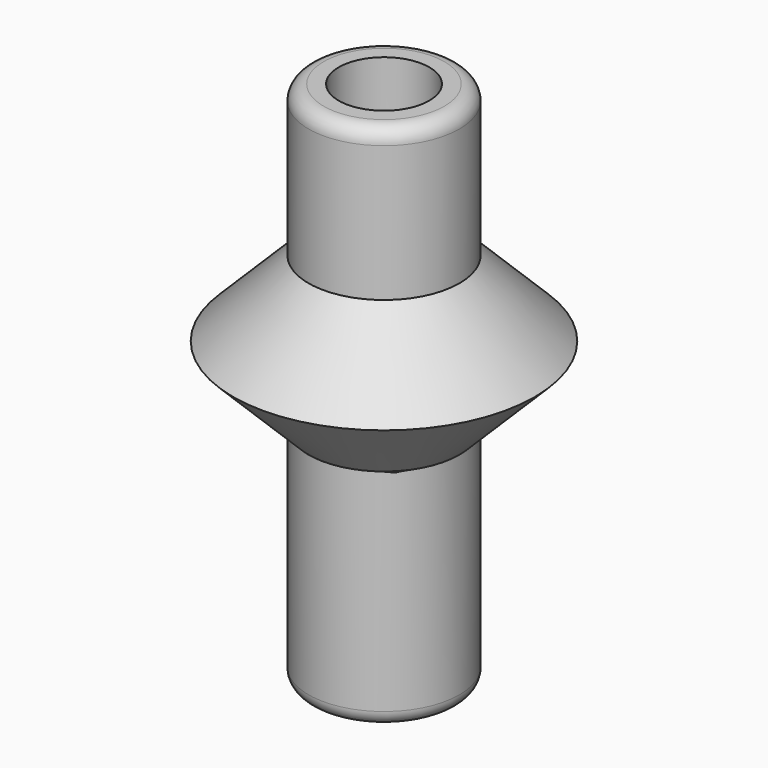
from build123d import *

# Parameters (mm, degrees)
F0_R         = 12.7
F1_DEPTH     = 38.1
F2_R         = 25.4
F2_R_2       = 12.7
F3_DEPTH     = 12.7
F4_R         = 2.54
F5_T1_DEPTH  = 10.7763073453
F5_T3_DEPTH  = 10.7763073453
F5_T9_DEPTH  = 23.4763073453
F5_S10_R     = 12.7
F5_T11_DEPTH = 14
F5_T15_DEPTH = 23.4763073453
F5_S16_R     = 12.7
F5_T17_DEPTH = 14
F5_T24_DEPTH = 23.4763073453
F5_S25_R     = 12.7
F5_T26_DEPTH = 14
F5_T30_DEPTH = 23.4763073453
F5_S31_R     = 12.7
F5_T32_DEPTH = 14
F5_T39_DEPTH = 23.4763073453
F5_S40_R     = 12.7
F5_T41_DEPTH = 14
F5_T45_DEPTH = 23.4763073453
F5_S46_R     = 12.7
F5_T47_DEPTH = 14
F5_T54_DEPTH = 23.4763073453
F5_S55_R     = 12.7
F5_T56_DEPTH = 14
F5_T60_DEPTH = 23.4763073453
F5_S61_R     = 12.7
F5_T62_DEPTH = 14
F8_R         = 12.7
F8_R_2       = 7.62
F9_DEPTH     = 25.4
F10_R        = 2.54
F11_DEPTH    = 25.4
F12_SIZE     = 12.69999


# Not quite as in the source:
# - a fillet or chamfer that OpenCascade refuses, or shapes differently, is made with other operations: its cross-section is extruded or revolved along the edge and cut away or added
# - a fillet or chamfer is up to 0.001 mm smaller than in the source, because OpenCascade refuses the exact size


with BuildPart() as f1:
    # F0 (on Top) → F1 (new body)
    with BuildSketch(Plane.XY):
        Circle(F0_R)
        with BuildLine():
            ThreePointArc((5.3881536726, 5.3881536726), (7.0399620377, 2.9160477546), (7.62, 0))
            ThreePointArc((7.62, 0), (7.0399620377, -2.9160477546), (5.3881536726, -5.3881536726))
            ThreePointArc((5.3881536726, -5.3881536726), (0, -7.62), (-5.3881536726, -5.3881536726))
            ThreePointArc((-5.3881536726, -5.3881536726), (-7.62, 0), (-5.3881536726, 5.3881536726))
            ThreePointArc((-5.3881536726, 5.3881536726), (0, 7.62), (5.3881536726, 5.3881536726))
        make_face(mode=Mode.SUBTRACT)
        with BuildLine():
            ThreePointArc((-5.3881536726, -5.3881536726), (0, -7.62), (5.3881536726, -5.3881536726))
            Line((5.3881536726, -5.3881536726), (-5.3881536726, -5.3881536726))
        make_face()
        with BuildLine():
            Line((-5.3881536726, -5.3881536726), (-5.3881536726, 5.3881536726))
            ThreePointArc((-5.3881536726, 5.3881536726), (-7.62, 0), (-5.3881536726, -5.3881536726))
        make_face()
        with BuildLine():
            ThreePointArc((5.3881536726, -5.3881536726), (7.0399620377, -2.9160477546), (7.62, 0))
            ThreePointArc((7.62, 0), (7.0399620377, 2.9160477546), (5.3881536726, 5.3881536726))
            Line((5.3881536726, 5.3881536726), (5.3881536726, -5.3881536726))
        make_face()
        with BuildLine():
            Line((-5.3881536726, 5.3881536726), (5.3881536726, 5.3881536726))
            ThreePointArc((5.3881536726, 5.3881536726), (0, 7.62), (-5.3881536726, 5.3881536726))
        make_face()
    extrude(amount=F1_DEPTH)

    # F4
    f4_edges = [f1.edges().sort_by_distance(p)[0] for p in [
        (-12.7, 0, 0),
    ]]
    fillet(f4_edges, radius=F4_R)

    # F5: fillet of radius 5.08 on 4 edges, made by hand

    # F5_s2 → F5_t1 (cut)
    with BuildSketch(Plane.XZ.offset(-5.3881536726)):
        with BuildLine():
            ThreePointArc((10.4681536726, 38.1), (6.8760512242, 36.6121024484), (5.3881536726, 33.02))
            Line((5.3881536726, 33.02), (5.3881536726, 38.1))
            Line((5.3881536726, 38.1), (10.4681536726, 38.1))
        make_face()
        with BuildLine():
            ThreePointArc((-10.4681536726, 38.1), (-6.8760512242, 36.6121024484), (-5.3881536726, 33.02))
            Line((-5.3881536726, 33.02), (-5.3881536726, 38.1))
            Line((-5.3881536726, 38.1), (-10.4681536726, 38.1))
        make_face()
    extrude(amount=F5_T1_DEPTH, mode=Mode.SUBTRACT)

    # F5_s4 → F5_t3 (cut)
    with BuildSketch(Plane.YZ.offset(-5.3881536726)):
        with BuildLine():
            ThreePointArc((-10.4681536726, 38.1), (-6.8760512242, 36.6121024484), (-5.3881536726, 33.02))
            Line((-5.3881536726, 33.02), (-5.3881536726, 38.1))
            Line((-5.3881536726, 38.1), (-10.4681536726, 38.1))
        make_face()
        with BuildLine():
            ThreePointArc((10.4681536726, 38.1), (6.8760512242, 36.6121024484), (5.3881536726, 33.02))
            Line((5.3881536726, 33.02), (5.3881536726, 38.1))
            Line((5.3881536726, 38.1), (10.4681536726, 38.1))
        make_face()
    extrude(amount=F5_T3_DEPTH, mode=Mode.SUBTRACT)


with BuildPart() as f3:
    # F2 (on face) → F3 (new body)
    with BuildSketch(Plane.XY.offset(38.1)):
        Circle(F2_R)
        Circle(F2_R_2, mode=Mode.SUBTRACT)
    extrude(amount=F3_DEPTH)

    # F6: F3 across face


with BuildPart() as f5_tool7:
    # F5_s8 → F5_t9 (new body)
    with BuildSketch(Plane.YZ.offset(-5.3881536726)):
        with BuildLine():
            ThreePointArc((10.4681536726, 38.1), (6.8760512242, 36.6121024484), (5.3881536726, 33.02))
            Line((5.3881536726, 33.02), (5.3881536726, 38.1))
            Line((5.3881536726, 38.1), (10.4681536726, 38.1))
        make_face()
    extrude(amount=F5_T9_DEPTH)

    # F5_s10 → F5_t11 (intersect, symmetric)
    with BuildSketch(Plane.XY.offset(35.6)):
        Circle(F5_S10_R)
    extrude(amount=F5_T11_DEPTH, both=True, mode=Mode.INTERSECT)

    split(bisect_by=Plane.YZ.offset(5.3881536726), keep=Keep.TOP)


with BuildPart() as f5_tool13:
    # F5_s14 → F5_t15 (new body)
    with BuildSketch(Plane.XZ.offset(-18.0881536726)):
        with BuildLine():
            ThreePointArc((10.4681536726, 38.1), (6.8760512242, 36.6121024484), (5.3881536726, 33.02))
            Line((5.3881536726, 33.02), (5.3881536726, 38.1))
            Line((5.3881536726, 38.1), (10.4681536726, 38.1))
        make_face()
    extrude(amount=F5_T15_DEPTH)

    # F5_s16 → F5_t17 (intersect, symmetric)
    with BuildSketch(Plane.XY.offset(35.6)):
        Circle(F5_S16_R)
    extrude(amount=F5_T17_DEPTH, both=True, mode=Mode.INTERSECT)

    split(bisect_by=Plane.XZ.offset(-5.3881536726), keep=Keep.BOTTOM)


with BuildPart() as f5_tool7_1:
    add(f5_tool7.part)

    # F5_t19: intersect F5_tool13
    add(f5_tool13.part, mode=Mode.INTERSECT)


with BuildPart() as f1_1:
    add(f1.part)

    # F5_t5: cut F5_tool7
    add(f5_tool7_1.part, mode=Mode.SUBTRACT)


with BuildPart() as f5_tool22:
    # F5_s23 → F5_t24 (new body)
    with BuildSketch(Plane.YZ.offset(18.0881536726)):
        with BuildLine():
            ThreePointArc((-10.4681536726, 38.1), (-6.8760512242, 36.6121024484), (-5.3881536726, 33.02))
            Line((-5.3881536726, 33.02), (-5.3881536726, 38.1))
            Line((-5.3881536726, 38.1), (-10.4681536726, 38.1))
        make_face()
    extrude(amount=-F5_T24_DEPTH)

    # F5_s25 → F5_t26 (intersect, symmetric)
    with BuildSketch(Plane.XY.offset(35.6)):
        Circle(F5_S25_R)
    extrude(amount=F5_T26_DEPTH, both=True, mode=Mode.INTERSECT)

    split(bisect_by=Plane.YZ.offset(5.3881536726), keep=Keep.TOP)


with BuildPart() as f5_tool28:
    # F5_s29 → F5_t30 (new body)
    with BuildSketch(Plane.XZ.offset(-5.3881536726)):
        with BuildLine():
            ThreePointArc((10.4681536726, 38.1), (6.8760512242, 36.6121024484), (5.3881536726, 33.02))
            Line((5.3881536726, 33.02), (5.3881536726, 38.1))
            Line((5.3881536726, 38.1), (10.4681536726, 38.1))
        make_face()
    extrude(amount=F5_T30_DEPTH)

    # F5_s31 → F5_t32 (intersect, symmetric)
    with BuildSketch(Plane.XY.offset(35.6)):
        Circle(F5_S31_R)
    extrude(amount=F5_T32_DEPTH, both=True, mode=Mode.INTERSECT)

    split(bisect_by=Plane.XZ.offset(5.3881536726), keep=Keep.TOP)


with BuildPart() as f5_tool22_1:
    add(f5_tool22.part)

    # F5_t34: intersect F5_tool28
    add(f5_tool28.part, mode=Mode.INTERSECT)


with BuildPart() as f1_2:
    add(f1_1.part)

    # F5_t20: cut F5_tool22
    add(f5_tool22_1.part, mode=Mode.SUBTRACT)


with BuildPart() as f5_tool37:
    # F5_s38 → F5_t39 (new body)
    with BuildSketch(Plane.YZ.offset(5.3881536726)):
        with BuildLine():
            ThreePointArc((-10.4681536726, 38.1), (-6.8760512242, 36.6121024484), (-5.3881536726, 33.02))
            Line((-5.3881536726, 33.02), (-5.3881536726, 38.1))
            Line((-5.3881536726, 38.1), (-10.4681536726, 38.1))
        make_face()
    extrude(amount=-F5_T39_DEPTH)

    # F5_s40 → F5_t41 (intersect, symmetric)
    with BuildSketch(Plane.XY.offset(35.6)):
        Circle(F5_S40_R)
    extrude(amount=F5_T41_DEPTH, both=True, mode=Mode.INTERSECT)

    split(bisect_by=Plane.YZ.offset(-5.3881536726), keep=Keep.BOTTOM)


with BuildPart() as f5_tool43:
    # F5_s44 → F5_t45 (new body)
    with BuildSketch(Plane.XZ.offset(18.0881536726)):
        with BuildLine():
            ThreePointArc((-10.4681536726, 38.1), (-6.8760512242, 36.6121024484), (-5.3881536726, 33.02))
            Line((-5.3881536726, 33.02), (-5.3881536726, 38.1))
            Line((-5.3881536726, 38.1), (-10.4681536726, 38.1))
        make_face()
    extrude(amount=-F5_T45_DEPTH)

    # F5_s46 → F5_t47 (intersect, symmetric)
    with BuildSketch(Plane.XY.offset(35.6)):
        Circle(F5_S46_R)
    extrude(amount=F5_T47_DEPTH, both=True, mode=Mode.INTERSECT)

    split(bisect_by=Plane.XZ.offset(5.3881536726), keep=Keep.TOP)


with BuildPart() as f5_tool37_1:
    add(f5_tool37.part)

    # F5_t49: intersect F5_tool43
    add(f5_tool43.part, mode=Mode.INTERSECT)


with BuildPart() as f1_3:
    add(f1_2.part)

    # F5_t35: cut F5_tool37
    add(f5_tool37_1.part, mode=Mode.SUBTRACT)


with BuildPart() as f5_tool52:
    # F5_s53 → F5_t54 (new body)
    with BuildSketch(Plane.XZ.offset(5.3881536726)):
        with BuildLine():
            ThreePointArc((-10.4681536726, 38.1), (-6.8760512242, 36.6121024484), (-5.3881536726, 33.02))
            Line((-5.3881536726, 33.02), (-5.3881536726, 38.1))
            Line((-5.3881536726, 38.1), (-10.4681536726, 38.1))
        make_face()
    extrude(amount=-F5_T54_DEPTH)

    # F5_s55 → F5_t56 (intersect, symmetric)
    with BuildSketch(Plane.XY.offset(35.6)):
        Circle(F5_S55_R)
    extrude(amount=F5_T56_DEPTH, both=True, mode=Mode.INTERSECT)

    split(bisect_by=Plane.XZ.offset(-5.3881536726), keep=Keep.BOTTOM)


with BuildPart() as f5_tool58:
    # F5_s59 → F5_t60 (new body)
    with BuildSketch(Plane.YZ.offset(-18.0881536726)):
        with BuildLine():
            ThreePointArc((10.4681536726, 38.1), (6.8760512242, 36.6121024484), (5.3881536726, 33.02))
            Line((5.3881536726, 33.02), (5.3881536726, 38.1))
            Line((5.3881536726, 38.1), (10.4681536726, 38.1))
        make_face()
    extrude(amount=F5_T60_DEPTH)

    # F5_s61 → F5_t62 (intersect, symmetric)
    with BuildSketch(Plane.XY.offset(35.6)):
        Circle(F5_S61_R)
    extrude(amount=F5_T62_DEPTH, both=True, mode=Mode.INTERSECT)

    split(bisect_by=Plane.YZ.offset(-5.3881536726), keep=Keep.BOTTOM)


with BuildPart() as f5_tool52_1:
    add(f5_tool52.part)

    # F5_t64: intersect F5_tool58
    add(f5_tool58.part, mode=Mode.INTERSECT)


with BuildPart() as f1_4:
    add(f1_3.part)

    # F5_t50: cut F5_tool52
    add(f5_tool52_1.part, mode=Mode.SUBTRACT)


with BuildPart() as f3_1:
    add(f3.part)
    add(f3.part.mirror(Plane.XY.offset(50.8)))

    # F12 (size 12.7 in the source; OpenCascade refuses exactly that, so slightly less here)
    f12_edges = [f3_1.edges().sort_by_distance(p)[0] for p in [
        (-25.4, 0, 38.1),
        (-25.4, 0, 63.5),
    ]]
    chamfer(f12_edges, length=F12_SIZE)


with BuildPart() as f9:
    # F8 (on offset) → F9 (new body)
    with BuildSketch(Plane.XY.offset(63.5)):
        Circle(F8_R)
        Circle(F8_R_2, mode=Mode.SUBTRACT)
    extrude(amount=F9_DEPTH)

    # F10
    f10_edges = [f9.edges().sort_by_distance(p)[0] for p in [
        (-12.7, 0, 88.9),
    ]]
    fillet(f10_edges, radius=F10_R)

    # F8 (on offset) → F11 (join)
    with BuildSketch(Plane.XY.offset(63.5)):
        Circle(F8_R)
        Circle(F8_R_2, mode=Mode.SUBTRACT)
    extrude(amount=-F11_DEPTH)


solid = Compound([f1_4.part, f3_1.part, f9.part])
